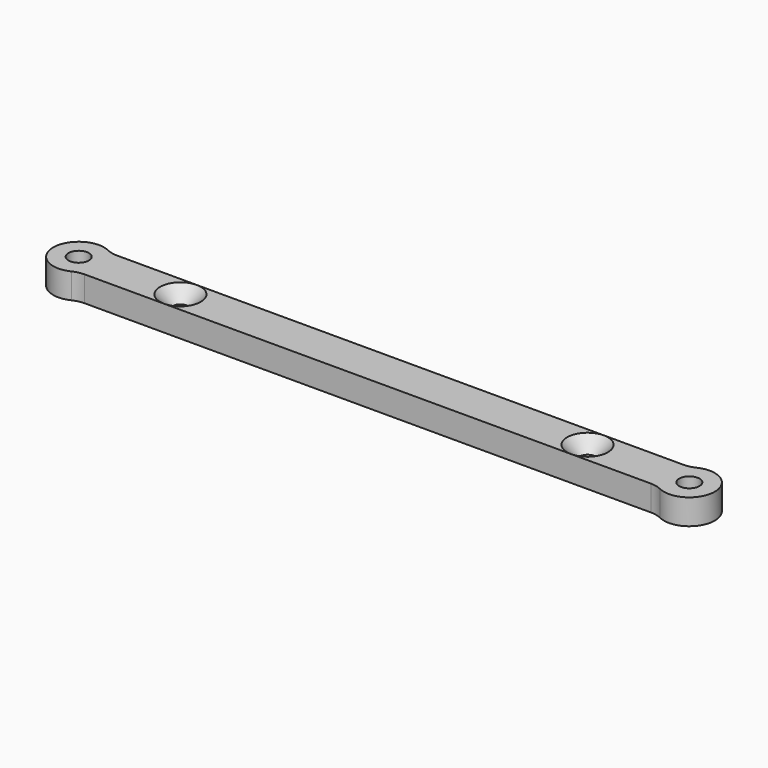
from build123d import *

# Parameters (mm, degrees)
F0_R     = 1.5
F0_R_2   = 2
F1_DEPTH = 5
F2_R     = 5
F3_SIZE2 = 2.49999
F3_SIZE  = 2.49999


# Not quite as in the source:
# - a fillet or chamfer is up to 0.001 mm smaller than in the source, because OpenCascade refuses the exact size


with BuildPart() as f1:
    # F0 (on Top) → F1 (new body)
    with BuildSketch(Plane.XY):
        with BuildLine():
            Line((57, 4), (0, 4))
            Line((0, 4), (0, -4))
            Line((0, -4), (57, -4))
            ThreePointArc((57, -4), (65, 0), (57, 4))
        make_face()
        with Locations((40, 0)):
            Circle(F0_R, mode=Mode.SUBTRACT)
        with Locations((60, 0)):
            Circle(F0_R_2, mode=Mode.SUBTRACT)
        with BuildLine():
            Line((0, 4), (-57, 4))
            ThreePointArc((-57, 4), (-65, 0), (-57, -4))
            Line((-57, -4), (0, -4))
            Line((0, -4), (0, 4))
        make_face()
        with Locations((-60, 0)):
            Circle(F0_R_2, mode=Mode.SUBTRACT)
        with Locations((-40, 0)):
            Circle(F0_R, mode=Mode.SUBTRACT)
    extrude(amount=F1_DEPTH)

    # F2
    f2_edges = [f1.edges().sort_by_distance(p)[0] for p in [
        (-57, 4, 2.5),
        (-57, -4, 2.5),
        (57, -4, 2.5),
        (57, 4, 2.5),
    ]]
    fillet(f2_edges, radius=F2_R)

    # F3 (size 2.5 and 2.5 in the source; OpenCascade refuses exactly that, so slightly less here)
    f3_edges = [f1.edges().sort_by_distance(p)[0] for p in [
        (38.5, 0, 5),
        (-41.5, 0, 5),
        (-62, 0, 0),
        (58, 0, 0),
    ]]
    chamfer(f3_edges, length=F3_SIZE, length2=F3_SIZE2)


solid = f1.part
